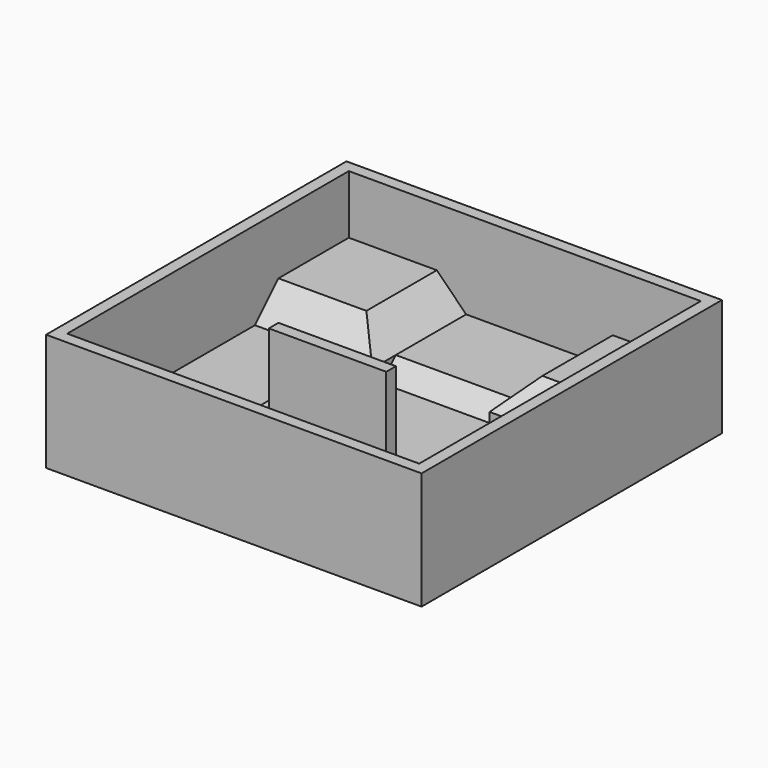
from build123d import *

# Parameters (mm, degrees)
F0_W      = 100
F0_H      = 100
F1_DEPTH  = 25
F2_W      = 100
F2_H      = 100
F3_DEPTH  = 50
F4_SIZE   = 24.99999
F4_2_SIZE = 24.99999
F4_3_SIZE = 24.99999
F4_4_SIZE = 24.99999
F4_5_SIZE = 24.99999
F4_6_SIZE = 24.99999
F4_7_SIZE = 24.99999
F4_8_SIZE = 24.99999
F6_DEPTH  = 100
F7_T      = -10
F8_W      = 100.09
F8_H      = 10.2765932679
F9_DEPTH  = 100


# Not quite as in the source:
# - a fillet or chamfer is up to 0.001 mm smaller than in the source, because OpenCascade refuses the exact size


with BuildPart() as f1:
    # F0 (on Top) → F1 (new body)
    with BuildSketch(Plane.XY):
        with Locations((150, 50)):
            Rectangle(F0_W, F0_H)
    extrude(amount=F1_DEPTH)

    # F4#7 (size 25 in the source; OpenCascade refuses exactly that, so slightly less here)
    f4_7_edges = [f1.edges().sort_by_distance(p)[0] for p in [
        (150, 0, 25),
    ]]
    chamfer(f4_7_edges, length=F4_7_SIZE)


with BuildPart() as f1b:
    # F0 (on Top) → F1, piece 2 (new body)
    with BuildSketch(Plane.XY):
        with Locations((50, -50)):
            Rectangle(F0_W, F0_H)
    extrude(amount=F1_DEPTH)

    # F4#6 (size 25 in the source; OpenCascade refuses exactly that, so slightly less here)
    f4_6_edges = [f1b.edges().sort_by_distance(p)[0] for p in [
        (100, -50, 25),
    ]]
    chamfer(f4_6_edges, length=F4_6_SIZE)


with BuildPart() as f1c:
    # F0 (on Top) → F1, piece 3 (new body)
    with BuildSketch(Plane.XY):
        with Locations((150, -150)):
            Rectangle(F0_W, F0_H)
    extrude(amount=F1_DEPTH)

    # F4#5 (size 25 in the source; OpenCascade refuses exactly that, so slightly less here)
    f4_5_edges = [f1c.edges().sort_by_distance(p)[0] for p in [
        (150, -100, 25),
    ]]
    chamfer(f4_5_edges, length=F4_5_SIZE)


with BuildPart() as f1d:
    # F0 (on Top) → F1, piece 4 (new body)
    with BuildSketch(Plane.XY):
        with Locations((250, -50)):
            Rectangle(F0_W, F0_H)
    extrude(amount=F1_DEPTH)

    # F4#8 (size 25 in the source; OpenCascade refuses exactly that, so slightly less here)
    f4_8_edges = [f1d.edges().sort_by_distance(p)[0] for p in [
        (200, -50, 25),
    ]]
    chamfer(f4_8_edges, length=F4_8_SIZE)


with BuildPart() as f3:
    # F2 (on face) → F3 (new body)
    with BuildSketch(Plane(origin=(0, 0, 0), x_dir=(1, 0, 0), z_dir=(0, 0, -1))):
        with Locations((50, -50)):
            Rectangle(F2_W, F2_H)
    extrude(amount=-F3_DEPTH)

    # F4#2 (size 25 in the source; OpenCascade refuses exactly that, so slightly less here)
    f4_2_edges = [f3.edges().sort_by_distance(p)[0] for p in [
        (50, 0, 50),
        (100, 50, 50),
    ]]
    chamfer(f4_2_edges, length=F4_2_SIZE)


with BuildPart() as f3b:
    # F2 (on face) → F3, piece 2 (new body)
    with BuildSketch(Plane(origin=(0, 0, 0), x_dir=(1, 0, 0), z_dir=(0, 0, -1))):
        with Locations((50, 150)):
            Rectangle(F2_W, F2_H)
    extrude(amount=-F3_DEPTH)

    # F4 (size 25 in the source; OpenCascade refuses exactly that, so slightly less here)
    f4_edges = [f3b.edges().sort_by_distance(p)[0] for p in [
        (100, -150, 50),
        (50, -100, 50),
    ]]
    chamfer(f4_edges, length=F4_SIZE)


with BuildPart() as f3c:
    # F2 (on face) → F3, piece 3 (new body)
    with BuildSketch(Plane(origin=(0, 0, 0), x_dir=(1, 0, 0), z_dir=(0, 0, -1))):
        with Locations((250, 150)):
            Rectangle(F2_W, F2_H)
    extrude(amount=-F3_DEPTH)

    # F4#4 (size 25 in the source; OpenCascade refuses exactly that, so slightly less here)
    f4_4_edges = [f3c.edges().sort_by_distance(p)[0] for p in [
        (250, -100, 50),
        (200, -150, 50),
    ]]
    chamfer(f4_4_edges, length=F4_4_SIZE)


with BuildPart() as f3d:
    # F2 (on face) → F3, piece 4 (new body)
    with BuildSketch(Plane(origin=(0, 0, 0), x_dir=(1, 0, 0), z_dir=(0, 0, -1))):
        with Locations((250, -50)):
            Rectangle(F2_W, F2_H)
    extrude(amount=-F3_DEPTH)

    # F4#3 (size 25 in the source; OpenCascade refuses exactly that, so slightly less here)
    f4_3_edges = [f3d.edges().sort_by_distance(p)[0] for p in [
        (200, 50, 50),
        (250, 0, 50),
    ]]
    chamfer(f4_3_edges, length=F4_3_SIZE)


with BuildPart() as f6:
    # F5 (on Top) → F6 (new body)
    with BuildSketch(Plane.XY):
        Polygon((-10, 110), (-10, 0), (-10, -210), (310, -210), (310, 110), align=None)
    extrude(amount=F6_DEPTH)

    # F7
    f7_openings = [f6.faces().sort_by_distance(p)[0] for p in [
        (150, -50, 100),
    ]]
    offset(amount=F7_T, openings=f7_openings)


with BuildPart() as f9:
    # F8 (on Top) → F9 (new body)
    with BuildSketch(Plane.XY):
        with Locations((150.1145795155, -105.1808483899)):
            Rectangle(F8_W, F8_H)
    extrude(amount=F9_DEPTH)


solid = Compound([f1.part, f1b.part, f1c.part, f1d.part, f3.part, f3b.part, f3c.part, f3d.part, f6.part, f9.part])
